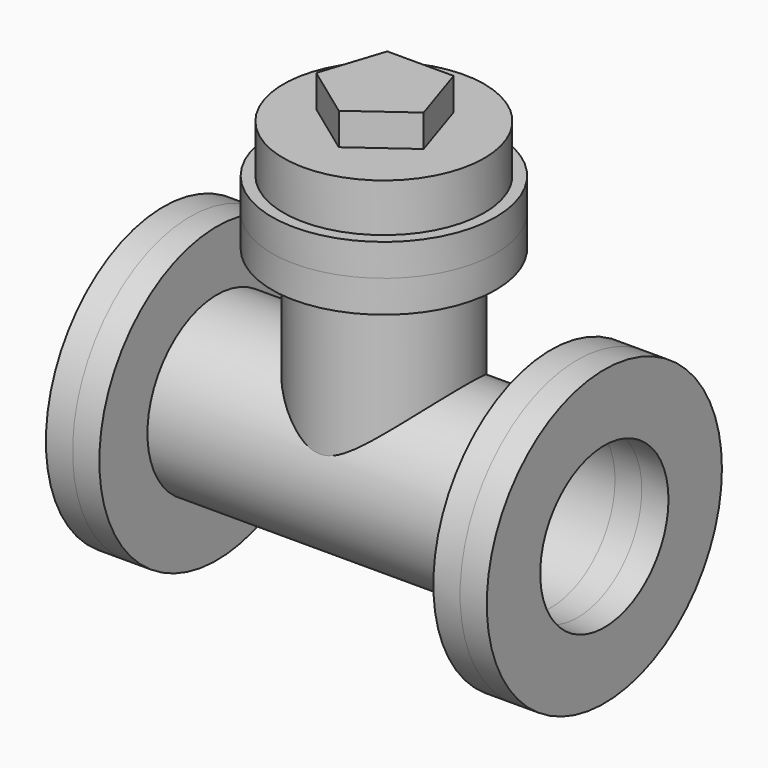
from build123d import *

# Parameters (mm, degrees)
F0_R      = 139.7
F0_R_2    = 76.2
F1_DEPTH  = 25.4
F3_R      = 139.7
F3_R_2    = 76.2
F4_DEPTH  = 25.4
F6_DEPTH  = 25.4
F7_DEPTH  = 25.4
F9_R      = 82.55
F9_R_2    = 76.2
F10_DEPTH = 317.5
F12_R     = 106.3625
F13_DEPTH = 30.48
F14_R     = 76.2
F15_REACH = 527.9471469057
F16_DEPTH = 30.48
F17_R     = 95.4249040927
F18_DEPTH = 45.72
F20_DEPTH = 30.48


with BuildPart() as f1:
    # F0 (on Right) → F1 (new body)
    with BuildSketch(Plane.YZ):
        Circle(F0_R)
        Circle(F0_R_2, mode=Mode.SUBTRACT)
    extrude(amount=F1_DEPTH)


with BuildPart() as f4:
    # F3 (on offset) → F4 (new body)
    with BuildSketch(Plane.YZ.offset(-317.5)):
        Circle(F3_R)
        Circle(F3_R_2, mode=Mode.SUBTRACT)
    extrude(amount=-F4_DEPTH)


with BuildPart() as f6:
    # F6 (new): a face of the model
    f6_faces = [f4.part.faces().sort_by_distance(p)[0] for p in [
        (-342.9, -135.7486873067, 0),
    ]]
    extrude(f6_faces, amount=F6_DEPTH)


with BuildPart() as f7:
    # F7 (new): a face of the model
    f7_faces = [f1.part.faces().sort_by_distance(p)[0] for p in [
        (25.4, -135.7486873067, 0),
    ]]
    extrude(f7_faces, amount=F7_DEPTH)


with BuildPart() as f1_1:
    add(f1.part)

    add(f4.part)  # F10 merges F4
    # F9 (on face) → F10 (join, through all)
    with BuildSketch(Plane.YZ.offset(-317.5)):
        Circle(F9_R)
        Circle(F9_R_2, mode=Mode.SUBTRACT)
    extrude(amount=F10_DEPTH)



with BuildPart() as f13:
    # F12 (on offset) → F13 (new body)
    with BuildSketch(Plane.XY.offset(203.2)):
        with Locations((-158.75, 0)):
            Circle(F12_R)
    extrude(amount=-F13_DEPTH)


with BuildPart() as f1_2:
    add(f1_1.part)

    add(f13.part)  # F15 merges F13
    f15_end = f1_2.faces().sort_by_distance((-158.75, -82.55, 0))[0]
    # F14 (on face) → F15 (join, up to a face of the model that its end follows)
    with BuildSketch(Plane(origin=(0, 0, 172.72), x_dir=(1, 0, 0), z_dir=(0, 0, -1))):
        with Locations((-158.75, 0)):
            Circle(F14_R)
    f15_long = extrude(amount=F15_REACH, mode=Mode.PRIVATE)
    add(split(f15_long, bisect_by=f15_end, keep=Keep.ALL, mode=Mode.PRIVATE).solids().sort_by_distance((-158.75, 0, 172.72))[0])


with BuildPart() as f16:
    # F16 (new): a face of the model
    f16_faces = [f1_2.part.faces().sort_by_distance(p)[0] for p in [
        (-158.75, 0, 203.2),
    ]]
    extrude(f16_faces, amount=F16_DEPTH)

    # F17 (on face) → F18 (join)
    with BuildSketch(Plane.XY.offset(233.68)):
        with Locations((-158.75, 0)):
            Circle(F17_R)
    extrude(amount=F18_DEPTH)

    # F19 (on face) → F20 (join)
    with BuildSketch(Plane.XY.offset(279.4)):
        Polygon((-127.2176910353, 43.4004999697), (-190.2823089647, 43.4004999697), (-209.7703476486, -16.5775158597), (-158.75, -53.6459682201), (-107.7296523514, -16.5775158597), align=None)
    extrude(amount=F20_DEPTH)


solid = Compound([f6.part, f7.part, f1_2.part, f16.part])
